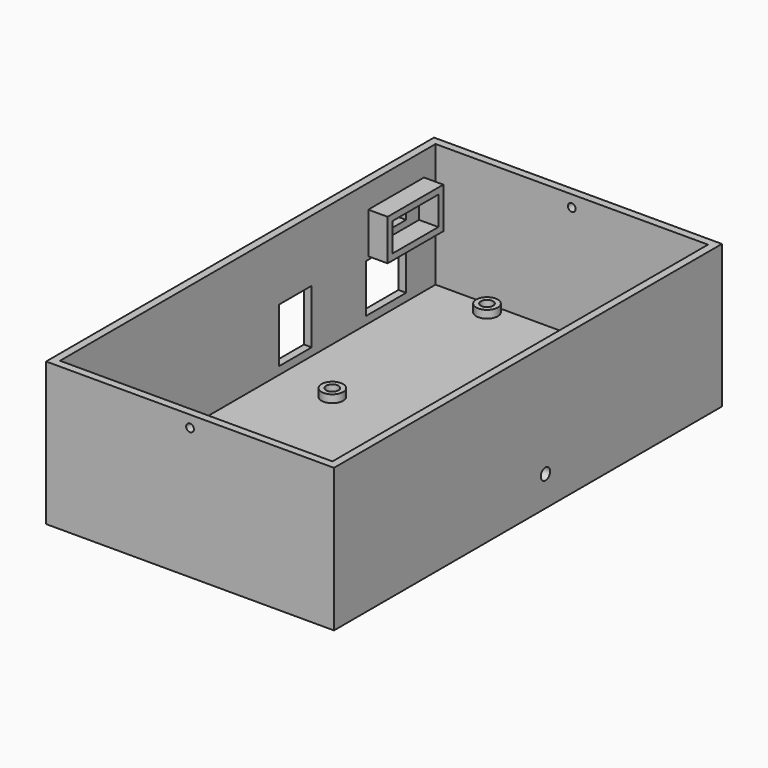
from build123d import *

# Parameters (mm, degrees)
F0_R      = 1.59
F1_DEPTH  = 5
F2_W      = 74.4103554785
F2_H      = 125.3275879622
F3_DEPTH  = 32
F4_R      = 2.7900010005
F4_R_2    = 2.7899997517
F4_R_3    = 2.79
F5_DEPTH  = 2
F6_DEPTH  = 37.001
F8_DEPTH  = 2.6
F9_W      = 13
F9_H      = 12.5
F9_W_2    = 10.5
F9_H_2    = 14.01349
F9_W_3    = 6.5
F9_H_3    = 4
F10_DEPTH = 3
F9_W_4    = 17.9999999672
F9_H_4    = 10.5999999672
F9_W_5    = 14.8
F9_H_5    = 7.4
F11_DEPTH = 7
F13_DEPTH = 6
F14_R     = 1
F15_DEPTH = 125.3285879622
F16_R     = 1.5
F17_DEPTH = 3


# Not quite as in the source:
# - a feature names something its author has since deleted; it is built from what else it names


with BuildPart() as f1:
    # F0 (on Top) → F1 (new body)
    with BuildSketch(Plane.XY):
        Polygon((27.9103554785, 29), (-46.5, 29), (-46.5, -29), (-46.5, -96.3275879622), (27.9103554785, -96.3275879622), align=None)
        with Locations((-30.1368717179, -24.2969288903)):
            Circle(F0_R, mode=Mode.SUBTRACT)
        with Locations((-28.8368717179, 24.0430711097)):
            Circle(F0_R, mode=Mode.SUBTRACT)
        with Locations((21.9631282821, -19.0569288903)):
            Circle(F0_R, mode=Mode.SUBTRACT)
        with Locations((21.9631282821, 8.8430711097)):
            Circle(F0_R, mode=Mode.SUBTRACT)
        with Locations((21.9631282821, -19.0569288903)):
            Circle(F0_R)
        with Locations((-28.8368717179, 24.0430711097)):
            Circle(F0_R)
        with Locations((-30.1368717179, -24.2969288903)):
            Circle(F0_R)
        with Locations((21.9631282821, 8.8430711097)):
            Circle(F0_R)
    extrude(amount=F1_DEPTH)

    # F2 (on face) → F3 (join)
    with BuildSketch(Plane.XY.offset(5)):
        with Locations((-9.2948222607, -33.6637939811)):
            Rectangle(F2_W, F2_H)
        Polygon((25.9103551507, 26.9999996722), (25.9103551507, -94.3275876343), (-44.4999996722, -94.3275876343), (-44.4999996722, -29), (-44.4999996722, 26.9999996722), align=None, mode=Mode.SUBTRACT)
    extrude(amount=F3_DEPTH)

    # F4 (on face) → F5 (join)
    with BuildSketch(Plane.XY.offset(5)):
        with Locations((-28.8368717179, 24.0430711097)):
            Circle(F4_R)
        with Locations((21.9631282821, 8.8430711097)):
            Circle(F4_R_2)
        with Locations((21.9631282821, -19.0569288903)):
            Circle(F4_R_3)
        with Locations((-30.1368717179, -24.2969288903)):
            Circle(F4_R_3)
    extrude(amount=F5_DEPTH)

    # F0 (on Top) → F6 (cut, through all)
    with BuildSketch(Plane.XY):
        with Locations((-30.1368717179, -24.2969288903)):
            Circle(F0_R)
        with Locations((21.9631282821, -19.0569288903)):
            Circle(F0_R)
        with Locations((21.9631282821, 8.8430711097)):
            Circle(F0_R)
        with Locations((-28.8368717179, 24.0430711097)):
            Circle(F0_R)
    extrude(amount=F6_DEPTH, mode=Mode.SUBTRACT)

    # F7 (on Top) → F8 (cut)
    with BuildSketch(Plane.XY):
        Polygon((-28.5388533662, -27.1075641711), (-26.9037809882, -24.3183220425), (-28.5017993398, -21.5076867618), (-31.7348900695, -21.4862936096), (-33.3699624476, -24.2755357382), (-31.7719440959, -27.0861710189), align=None)
        Polygon((23.649281557, -21.8155916945), (25.1952769884, -18.9760087217), (23.5091237135, -16.2173459175), (20.2769750072, -16.2982660862), (18.7309795758, -19.137849059), (20.4171328507, -21.8965118631), align=None)
        Polygon((23.5751015985, 6.040416054), (25.1962854165, 8.837753424), (23.5843121002, 11.6404084796), (20.3511549658, 11.6457261653), (18.7299711478, 8.8483887953), (20.3419444641, 6.0457337397), align=None)
        Polygon((-28.8368717179, 20.8099096022), (-26.0368717179, 22.4264903559), (-26.0368717179, 25.6596518634), (-28.8368717179, 27.2762326171), (-31.6368717179, 25.6596518634), (-31.6368717179, 22.4264903559), align=None)
    extrude(amount=F8_DEPTH, mode=Mode.SUBTRACT)

    # F9 (on face) → F10 (cut)
    with BuildSketch(Plane(origin=(-46.5, 0, 0), x_dir=(0, -1, 0), z_dir=(-1, 0, 0))):
        with Locations((-11.010112679, 13.25)):
            Rectangle(F9_W, F9_H)
        with Locations((18.2770747468, 14.006745)):
            Rectangle(F9_W_2, F9_H_2)
        with Locations((-14.260112679, 25.6000000164)):
            Rectangle(F9_W_3, F9_H_3)
    extrude(amount=-F10_DEPTH, mode=Mode.SUBTRACT)

    # F9 (on face) → F11 (join)
    with BuildSketch(Plane(origin=(-46.5, 0, 0), x_dir=(0, -1, 0), z_dir=(-1, 0, 0))):
        with Locations((-14.260112679, 25.6000000164)):
            Rectangle(F9_W_4, F9_H_4)
        with Locations((-14.260112679, 25.6000000164)):
            Rectangle(F9_W_5, F9_H_5, mode=Mode.SUBTRACT)
    extrude(amount=-F11_DEPTH)

    # F12 (on face) → F13 (cut)
    with BuildSketch(Plane.XY.offset(5)):
        with BuildLine():
            ThreePointArc((-40.7473873347, 2.5), (-41.9973873347, 1.25), (-40.7473873347, 0))
            Line((-40.7473873347, 0), (-10.7473873347, 0))
            ThreePointArc((-10.7473873347, 0), (-9.4973873347, 1.25), (-10.7473873347, 2.5))
            Line((-10.7473873347, 2.5), (-40.7473873347, 2.5))
        make_face()
        with BuildLine():
            ThreePointArc((-40.7473873347, -2.0948293991), (-41.9973873347, -3.3448293991), (-40.7473873347, -4.5948293991))
            Line((-40.7473873347, -4.5948293991), (-10.7473873347, -4.5948293991))
            ThreePointArc((-10.7473873347, -4.5948293991), (-9.4973873347, -3.3448293991), (-10.7473873347, -2.0948293991))
            Line((-10.7473873347, -2.0948293991), (-40.7473873347, -2.0948293991))
        make_face()
        with BuildLine():
            ThreePointArc((-40.7473873347, -6.6774361208), (-41.9973873347, -7.9274361208), (-40.7473873347, -9.1774361208))
            Line((-40.7473873347, -9.1774361208), (-10.7473873347, -9.1774361208))
            ThreePointArc((-10.7473873347, -9.1774361208), (-9.4973873347, -7.9274361208), (-10.7473873347, -6.6774361208))
            Line((-10.7473873347, -6.6774361208), (-40.7473873347, -6.6774361208))
        make_face()
        with BuildLine():
            ThreePointArc((-40.7473873347, -11.2855438516), (-41.9973873347, -12.5355438516), (-40.7473873347, -13.7855438516))
            Line((-40.7473873347, -13.7855438516), (-10.7473873347, -13.7855438516))
            ThreePointArc((-10.7473873347, -13.7855438516), (-9.4973873347, -12.5355438516), (-10.7473873347, -11.2855438516))
            Line((-10.7473873347, -11.2855438516), (-40.7473873347, -11.2855438516))
        make_face()
        with BuildLine():
            ThreePointArc((-40.7473873347, -15.9455886483), (-41.9973873347, -17.1955886483), (-40.7473873347, -18.4455886483))
            Line((-40.7473873347, -18.4455886483), (-10.7473873347, -18.4455886483))
            ThreePointArc((-10.7473873347, -18.4455886483), (-9.4973873347, -17.1955886483), (-10.7473873347, -15.9455886483))
            Line((-10.7473873347, -15.9455886483), (-40.7473873347, -15.9455886483))
        make_face()
        with BuildLine():
            ThreePointArc((-40.7473873347, 6.6440958157), (-41.9973873347, 5.3940958157), (-40.7473873347, 4.1440958157))
            Line((-40.7473873347, 4.1440958157), (-10.7473873347, 4.1440958157))
            ThreePointArc((-10.7473873347, 4.1440958157), (-9.4973873347, 5.3940958157), (-10.7473873347, 6.6440958157))
            Line((-10.7473873347, 6.6440958157), (-40.7473873347, 6.6440958157))
        make_face()
        with BuildLine():
            ThreePointArc((-40.7473873347, 11.013558656), (-41.9973873347, 9.763558656), (-40.7473873347, 8.513558656))
            Line((-40.7473873347, 8.513558656), (-10.7473873347, 8.513558656))
            ThreePointArc((-10.7473873347, 8.513558656), (-9.4973873347, 9.763558656), (-10.7473873347, 11.013558656))
            Line((-10.7473873347, 11.013558656), (-40.7473873347, 11.013558656))
        make_face()
        with BuildLine():
            ThreePointArc((-40.7473873347, 15.4895936698), (-41.9973873347, 14.2395936698), (-40.7473873347, 12.9895936698))
            Line((-40.7473873347, 12.9895936698), (-10.7473873347, 12.9895936698))
            ThreePointArc((-10.7473873347, 12.9895936698), (-9.4973873347, 14.2395936698), (-10.7473873347, 15.4895936698))
            Line((-10.7473873347, 15.4895936698), (-40.7473873347, 15.4895936698))
        make_face()
        with BuildLine():
            ThreePointArc((-40.7473873347, 19.7524824739), (-41.9973873347, 18.5024824739), (-40.7473873347, 17.2524824739))
            Line((-40.7473873347, 17.2524824739), (-10.7473873347, 17.2524824739))
            ThreePointArc((-10.7473873347, 17.2524824739), (-9.4973873347, 18.5024824739), (-10.7473873347, 19.7524824739))
            Line((-10.7473873347, 19.7524824739), (-40.7473873347, 19.7524824739))
        make_face()
    extrude(amount=F13_DEPTH, mode=Mode.SUBTRACT)

    # F14 (on face) → F15 (cut, through all)
    with BuildSketch(Plane.XZ.offset(96.3275879622)):
        with Locations((-9.2948222607, 34)):
            Circle(F14_R)
    extrude(amount=-F15_DEPTH, mode=Mode.SUBTRACT)

    # F16 (on face) → F17 (cut)
    with BuildSketch(Plane.YZ.offset(27.9103554785)):
        with Locations((-27.9986988753, 7.8254723921)):
            Circle(F16_R)
    extrude(amount=-F17_DEPTH, mode=Mode.SUBTRACT)


solid = f1.part
